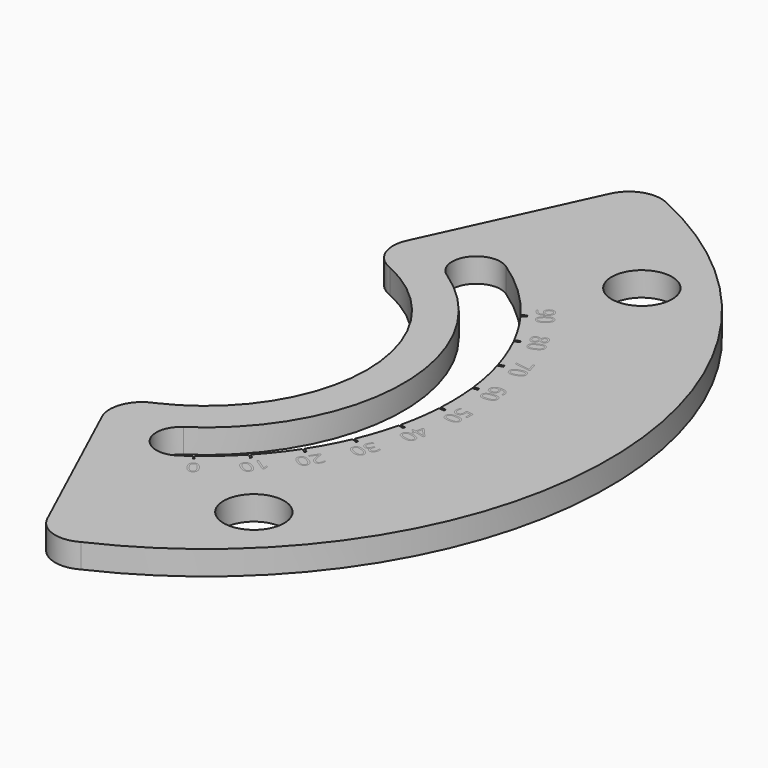
from build123d import *

# Parameters (mm, degrees)
F2_DEPTH       = 3
F0_R           = 3.75
F3_DEPTH       = 25
F5_DEPTH       = 25
F7_DEPTH       = 0.1
F8_TEXT_SIZE   = 2.5893459204
F8_TEXT_SIZE_2 = 2.5559105431
F9_DEPTH       = 0.1
F10_DEPTH      = 0.1


# Not quite as in the source:
# - a feature names something its author has since deleted; it is built from what else it names
# - Text() gives the source's letters only with a copy of the font that has no kerning and outlines rounded to 1/6400 em; it was checked with that copy


with BuildPart() as f2:
    # F1 (on Top) → F2 (new body)
    with BuildSketch(Plane.XY):
        with BuildLine():
            Line((15.3002332561, 43.6149479969), (6.0775941037, 23.6094971738))
            ThreePointArc((6.0775941037, 23.6094971738), (6.0202884054, 20.3905792849), (8.3532666321, 18.1720372158))
            ThreePointArc((8.3532666321, 18.1720372158), (20, 0), (8.3532666321, -18.1720372158))
            ThreePointArc((8.3532666321, -18.1720372158), (6.0202884054, -20.3905792849), (6.0775941037, -23.6094971738))
            Line((6.0775941037, -23.6094971738), (15.3002332561, -43.6149479969))
            ThreePointArc((15.3002332561, -43.6149479969), (17.7077688734, -45.7481016038), (20.9074878909, -45.4189052058))
            ThreePointArc((20.9074878909, -45.4189052058), (50, 0), (20.9074878909, 45.4189052058))
            ThreePointArc((20.9074878909, 45.4189052058), (17.7077688734, 45.7481016038), (15.3002332561, 43.6149479969))
        make_face()
    extrude(amount=F2_DEPTH)

    # F0 (on Top) → F3 (cut)
    with BuildSketch(Plane.XY):
        with Locations((30.0520382004, 30.0520382004)):
            Circle(F0_R)
        with Locations((30.0520382004, -30.0520382004)):
            Circle(F0_R)
    extrude(amount=F3_DEPTH, mode=Mode.SUBTRACT)

    # F4 (on face) → F5 (cut)
    with BuildSketch(Plane.XY.offset(3)):
        with BuildLine():
            ThreePointArc((16.9171135648, 25.402394939), (12.7572667263, 24.5683240307), (13.5913376346, 20.4084771921))
            ThreePointArc((13.5913376346, 20.4084771921), (24.52, 0), (13.5913376346, -20.4084771921))
            ThreePointArc((13.5913376346, -20.4084771921), (12.7572667263, -24.5683240307), (16.9171135648, -25.402394939))
            ThreePointArc((16.9171135648, -25.402394939), (30.52, 0), (16.9171135648, 25.402394939))
        make_face()
    extrude(amount=-F5_DEPTH, mode=Mode.SUBTRACT)

    # F6 (on face) → F7 (cut)
    with BuildSketch(Plane.XY.offset(3)):
        with BuildLine():
            Line((22.3245326851, -20.8107097523), (21.8424331722, -20.3575135713))
            Line((21.8424331722, -20.3575135713), (21.6712100752, -20.539656703))
            Line((21.6712100752, -20.539656703), (22.1533263244, -20.9928686169))
            ThreePointArc((22.1533263244, -20.9928686169), (22.2391160116, -20.9019644776), (22.3245326851, -20.8107097523))
        make_face()
        with BuildLine():
            Line((22.8029082553, -21.2604052523), (22.3245326851, -20.8107097523))
            ThreePointArc((22.3245326851, -20.8107097523), (22.2391160116, -20.9019644776), (22.1533263244, -20.9928686169))
            Line((22.1533263244, -20.9928686169), (22.6316851583, -21.4425483839))
            Line((22.6316851583, -21.4425483839), (22.8029082553, -21.2604052523))
        make_face()
        with BuildLine():
            Line((24.9011606776, -16.4757713175), (25.4544869851, -16.8386309516))
            ThreePointArc((25.4544869851, -16.8386309516), (25.5232354691, -16.7342418768), (25.5915558551, -16.6295721207))
            Line((25.5915558551, -16.6295721207), (25.0382487559, -16.266725083))
            Line((25.0382487559, -16.266725083), (24.9011606776, -16.4757713175))
        make_face()
        with BuildLine():
            ThreePointArc((25.5915558551, -16.6295721207), (25.5232354691, -16.7342418768), (25.4544869851, -16.8386309516))
            Line((25.4544869851, -16.8386309516), (26.0035008955, -17.1986626073))
            Line((26.0035008955, -17.1986626073), (26.1405889738, -16.9896163727))
            Line((26.1405889738, -16.9896163727), (25.5915558551, -16.6295721207))
        make_face()
        with BuildLine():
            Line((27.3784293363, -11.9138763918), (27.9862404287, -12.1754156672))
            ThreePointArc((27.9862404287, -12.1754156672), (28.0358696639, -12.0606970026), (28.0850286571, -11.9457760455))
            Line((28.0850286571, -11.9457760455), (27.4772386644, -11.6842458493))
            Line((27.4772386644, -11.6842458493), (27.3784293363, -11.9138763918))
        make_face()
        with BuildLine():
            ThreePointArc((28.0850286571, -11.9457760455), (28.0358696639, -12.0606970026), (27.9862404287, -12.1754156672))
            Line((27.9862404287, -12.1754156672), (28.589314492, -12.4349166132))
            Line((28.589314492, -12.4349166132), (28.6881238202, -12.2052860708))
            Line((28.6881238202, -12.2052860708), (28.0850286571, -11.9457760455))
        make_face()
        with BuildLine():
            Line((29.0281361926, -6.9918633271), (29.6720598968, -7.1441767533))
            ThreePointArc((29.6720598968, -7.1441767533), (29.7010697512, -7.022596075), (29.7295814335, -6.9008976076))
            Line((29.7295814335, -6.9008976076), (29.0856800827, -6.7485894689))
            Line((29.0856800827, -6.7485894689), (29.0281361926, -6.9918633271))
        make_face()
        with BuildLine():
            ThreePointArc((29.7295814335, -6.9008976076), (29.7010697512, -7.022596075), (29.6720598968, -7.1441767533))
            Line((29.6720598968, -7.1441767533), (30.3109651251, -7.2953031113))
            Line((30.3109651251, -7.2953031113), (30.3685090151, -7.0520292531))
            Line((30.3685090151, -7.0520292531), (29.7295814335, -6.9008976076))
        make_face()
        with BuildLine():
            Line((29.8004159178, -1.8585087371), (30.4609884927, -1.8969923694))
            ThreePointArc((30.4609884927, -1.8969923694), (30.4685020918, -1.77222467), (30.4755046467, -1.6474272453))
            Line((30.4755046467, -1.6474272453), (29.8149550032, -1.608944949))
            Line((29.8149550032, -1.608944949), (29.8004159178, -1.8585087371))
        make_face()
        with BuildLine():
            Line((29.6719249814, 3.3310225904), (30.329179444, 3.4075319884))
            ThreePointArc((30.329179444, 3.4075319884), (30.3149696759, 3.531715383), (30.3002514388, 3.6558395405))
            Line((30.3002514388, 3.6558395405), (29.6430197923, 3.5793327985))
            Line((29.6430197923, 3.5793327985), (29.6719249814, 3.3310225904))
        make_face()
        with BuildLine():
            ThreePointArc((30.3002514388, 3.6558395405), (30.3149696759, 3.531715383), (30.329179444, 3.4075319884))
            Line((30.329179444, 3.4075319884), (30.9813115363, 3.4834451037))
            Line((30.9813115363, 3.4834451037), (30.9524063472, 3.7317553118))
            Line((30.9524063472, 3.7317553118), (30.3002514388, 3.6558395405))
        make_face()
        with BuildLine():
            ThreePointArc((30.4755046467, -1.6474272453), (30.4685020918, -1.77222467), (30.4609884927, -1.8969923694))
            Line((30.4609884927, -1.8969923694), (31.1164128372, -1.9351760761))
            Line((31.1164128372, -1.9351760761), (31.1309519226, -1.6856122879))
            Line((31.1309519226, -1.6856122879), (30.4755046467, -1.6474272453))
        make_face()
        with BuildLine():
            Line((28.6465472509, 8.4198678259), (29.2806169142, 8.6090576212))
            ThreePointArc((29.2806169142, 8.6090576212), (29.2451132944, 8.7289030466), (29.2091191502, 8.8486020631))
            Line((29.2091191502, 8.8486020631), (28.5750714982, 8.6594188354))
            Line((28.5750714982, 8.6594188354), (28.6465472509, 8.4198678259))
        make_face()
        with BuildLine():
            ThreePointArc((29.2091191502, 8.8486020631), (29.2451132944, 8.7289030466), (29.2806169142, 8.6090576212))
            Line((29.2806169142, 8.6090576212), (29.9097448999, 8.7967729494))
            Line((29.9097448999, 8.7967729494), (29.8382691472, 9.0363239588))
            Line((29.8382691472, 9.0363239588), (29.2091191502, 8.8486020631))
        make_face()
        with BuildLine():
            ThreePointArc((27.3469955736, 13.5503591501), (27.2912712624, 13.6622440647), (27.2350891981, 13.7738998243))
            Line((27.2350891981, 13.7738998243), (26.6433907604, 13.4777585109))
            Line((26.6433907604, 13.4777585109), (26.7552765948, 13.254207556))
            Line((26.7552765948, 13.254207556), (27.3469955736, 13.5503591501))
        make_face()
        with BuildLine():
            Line((27.8222171043, 14.0677536157), (27.2350891981, 13.7738998243))
            ThreePointArc((27.2350891981, 13.7738998243), (27.2912712624, 13.6622440647), (27.3469955736, 13.5503591501))
            Line((27.3469955736, 13.5503591501), (27.9341029387, 13.8442026608))
            Line((27.9341029387, 13.8442026608), (27.8222171043, 14.0677536157))
        make_face()
        with BuildLine():
            Line((18.576182603, -24.8380434693), (18.2806165931, -24.4395060707))
            ThreePointArc((18.2806165931, -24.4395060707), (18.1803669946, -24.5141725527), (18.0798124273, -24.5884278186))
            Line((18.0798124273, -24.5884278186), (18.3753784373, -24.9869652173))
            Line((18.3753784373, -24.9869652173), (18.576182603, -24.8380434693))
        make_face()
        with BuildLine():
            ThreePointArc((18.0798124273, -24.5884278186), (18.1803669946, -24.5141725527), (18.2806165931, -24.4395060707))
            Line((18.2806165931, -24.4395060707), (17.8866106231, -23.9082334985))
            Line((17.8866106231, -23.9082334985), (17.7862085402, -23.9826943725))
            Line((17.7862085402, -23.9826943725), (17.6858064573, -24.0571552465))
            Line((17.6858064573, -24.0571552465), (18.0798124273, -24.5884278186))
        make_face()
        with BuildLine():
            Line((24.9651889831, 18.6739603574), (24.4378301548, 18.2828569246))
            ThreePointArc((24.4378301548, 18.2828569246), (24.512501936, 18.1826194163), (24.5867625722, 18.0820769332))
            Line((24.5867625722, 18.0820769332), (25.1141029505, 18.4731666829))
            Line((25.1141029505, 18.4731666829), (24.9651889831, 18.6739603574))
        make_face()
        with BuildLine():
            ThreePointArc((24.5867625722, 18.0820769332), (24.512501936, 18.1826194163), (24.4378301548, 18.2828569246))
            Line((24.4378301548, 18.2828569246), (23.9063660708, 17.8887089243))
            Line((23.9063660708, 17.8887089243), (24.0552800382, 17.6879152499))
            Line((24.0552800382, 17.6879152499), (24.5867625722, 18.0820769332))
        make_face()
    extrude(amount=-F7_DEPTH, mode=Mode.SUBTRACT)

    # F8 (on face) → F9 (cut)
    with BuildSketch(Plane.XY.offset(3)):
        with Locations(Location((24.0622166206, -20.7506507427), (0, 0, -123.4383782973))):
            Text('10', F8_TEXT_SIZE, font='Open Sans', text_align=(TextAlign.LEFT, TextAlign.BOTTOM))
        with Locations(Location((27.5298860922, -16.3815558403), (0, 0, -123.4383782973))):
            Text('20', F8_TEXT_SIZE, font='Open Sans', text_align=(TextAlign.LEFT, TextAlign.BOTTOM))
        with Locations(Location((29.9562725822, -11.3521686466), (0, 0, -113.4383782973))):
            Text('30', F8_TEXT_SIZE, font='Open Sans', text_align=(TextAlign.LEFT, TextAlign.BOTTOM))
        with Locations(Location((31.4724528883, -5.9778515531), (0, 0, -103.4383782973))):
            Text('40', F8_TEXT_SIZE, font='Open Sans', text_align=(TextAlign.LEFT, TextAlign.BOTTOM))
        with Locations(Location((32.0323586393, -0.4219004651), (0, 0, -93.4383782973))):
            Text('50', F8_TEXT_SIZE, font='Open Sans', text_align=(TextAlign.LEFT, TextAlign.BOTTOM))
        with Locations(Location((31.6189773822, 5.1468698551), (0, 0, -83.4383782973))):
            Text('60', F8_TEXT_SIZE, font='Open Sans', text_align=(TextAlign.LEFT, TextAlign.BOTTOM))
        with Locations(Location((30.2448694973, 10.5592551391), (0, 0, -73.4383782973))):
            Text('70', F8_TEXT_SIZE, font='Open Sans', text_align=(TextAlign.LEFT, TextAlign.BOTTOM))
        with Locations(Location((27.9517865573, 15.650802799), (0, 0, -63.4383782973))):
            Text('80', F8_TEXT_SIZE, font='Open Sans', text_align=(TextAlign.LEFT, TextAlign.BOTTOM))
        with Locations(Location((24.8094027271, 20.2668087355), (0, 0, -53.4383782973))):
            Text('90', F8_TEXT_SIZE, font='Open Sans', text_align=(TextAlign.LEFT, TextAlign.BOTTOM))
        with Locations(Location((19.6643962398, -25.2561679699), (0, 0, -143.4383782973))):
            Text('0', F8_TEXT_SIZE_2, font='Open Sans', text_align=(TextAlign.LEFT, TextAlign.BOTTOM))
    extrude(amount=-F9_DEPTH, mode=Mode.SUBTRACT)


with BuildPart() as f10:
    # F8 (on face) → F10 (new body)
    with BuildSketch(Plane.XY.offset(3)):
        with Locations(Location((24.0622166206, -20.7506507427), (0, 0, -123.4383782973))):
            Text('10', F8_TEXT_SIZE, font='Open Sans', text_align=(TextAlign.LEFT, TextAlign.BOTTOM))
        with Locations(Location((27.5298860922, -16.3815558403), (0, 0, -123.4383782973))):
            Text('20', F8_TEXT_SIZE, font='Open Sans', text_align=(TextAlign.LEFT, TextAlign.BOTTOM))
        with Locations(Location((29.9562725822, -11.3521686466), (0, 0, -113.4383782973))):
            Text('30', F8_TEXT_SIZE, font='Open Sans', text_align=(TextAlign.LEFT, TextAlign.BOTTOM))
        with Locations(Location((31.4724528883, -5.9778515531), (0, 0, -103.4383782973))):
            Text('40', F8_TEXT_SIZE, font='Open Sans', text_align=(TextAlign.LEFT, TextAlign.BOTTOM))
        with Locations(Location((32.0323586393, -0.4219004651), (0, 0, -93.4383782973))):
            Text('50', F8_TEXT_SIZE, font='Open Sans', text_align=(TextAlign.LEFT, TextAlign.BOTTOM))
        with Locations(Location((31.6189773822, 5.1468698551), (0, 0, -83.4383782973))):
            Text('60', F8_TEXT_SIZE, font='Open Sans', text_align=(TextAlign.LEFT, TextAlign.BOTTOM))
        with Locations(Location((30.2448694973, 10.5592551391), (0, 0, -73.4383782973))):
            Text('70', F8_TEXT_SIZE, font='Open Sans', text_align=(TextAlign.LEFT, TextAlign.BOTTOM))
        with Locations(Location((27.9517865573, 15.650802799), (0, 0, -63.4383782973))):
            Text('80', F8_TEXT_SIZE, font='Open Sans', text_align=(TextAlign.LEFT, TextAlign.BOTTOM))
        with Locations(Location((24.8094027271, 20.2668087355), (0, 0, -53.4383782973))):
            Text('90', F8_TEXT_SIZE, font='Open Sans', text_align=(TextAlign.LEFT, TextAlign.BOTTOM))
        with Locations(Location((19.6643962398, -25.2561679699), (0, 0, -143.4383782973))):
            Text('0', F8_TEXT_SIZE_2, font='Open Sans', text_align=(TextAlign.LEFT, TextAlign.BOTTOM))
    extrude(amount=-F10_DEPTH)


solid = Compound([f2.part, f10.part])
